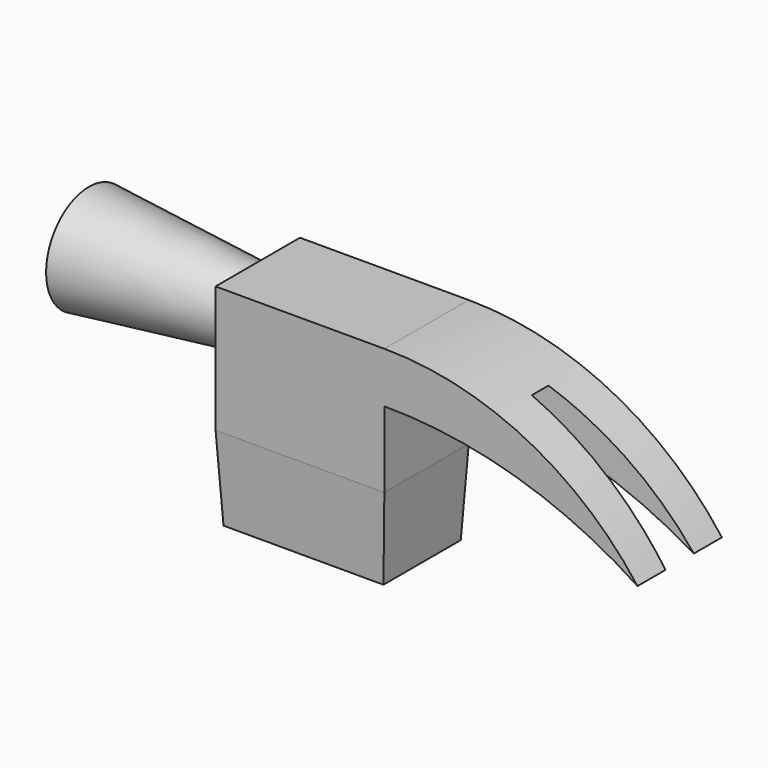
from build123d import *

# Parameters (mm, degrees)
F0_W       = 40
F0_H       = 29.999999
F1_DEPTH   = 12.5
F2_R       = 8.5
F3_DEPTH   = 40
F3_TAPER   = -6
F5_DEPTH   = 12.5
F1_FACE1_W = 40
F1_FACE1_H = 25
F6_DEPTH   = 20
F6_TAPER   = 3
F8_DEPTH   = 25


with BuildPart() as f1:
    # F0 (on Front) → F1 (new body, symmetric)
    with BuildSketch(Plane.XZ):
        with Locations((0, 14.999999)):
            Rectangle(F0_W, F0_H)
    extrude(amount=F1_DEPTH, both=True)

    # F2 (on face) → F3 (join)
    with BuildSketch(Plane(origin=(-20, 0, 0), x_dir=(0, -1, 0), z_dir=(-1, 0, 0))):
        with Locations((0, 20)):
            Circle(F2_R)
    extrude(amount=F3_DEPTH, taper=F3_TAPER)

    # F4 (on Front) → F5 (join, symmetric)
    with BuildSketch(Plane.XZ):
        with BuildLine():
            ThreePointArc((20, 18), (51.32092, 13.403065), (80, 0))
            ThreePointArc((80, 0), (53.54102, 22.082039), (20, 30))
            Line((20, 30), (20, 18))
        make_face()
    extrude(amount=F5_DEPTH, both=True)

    # F7 (on Top) → F8 (cut)
    with BuildSketch(Plane.XY):
        Polygon((98.108158, 5.141631), (30, 1.572233), (30, -1.572233), (98.108158, -5.141631), align=None)
    extrude(amount=F8_DEPTH, mode=Mode.SUBTRACT)


with BuildPart() as f6:
    # F1_face1 (on face) → F6 (new body)
    with BuildSketch(Plane(origin=(0, 0, 0), x_dir=(1, 0, 0), z_dir=(0, 0, -1))):
        Rectangle(F1_FACE1_W, F1_FACE1_H)
    extrude(amount=F6_DEPTH, taper=F6_TAPER)


solid = Compound([f1.part, f6.part])
